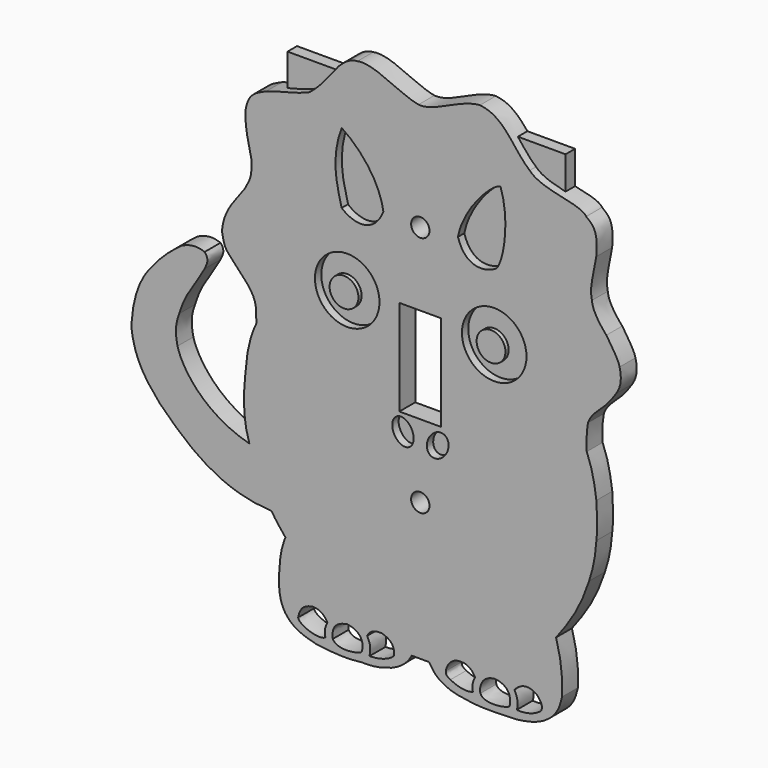
from build123d import *

# Parameters (mm, degrees)
F0_R     = 8.1256279654
F1_DEPTH = 5
F2_W     = 10.541
F2_H     = 24.0792
F2_R     = 2.3114
F3_DEPTH = 25
F2_R_2   = 8.1256279654
F4_DEPTH = 3
F5_DEPTH = 3
F6_R     = 3.6295881973
F7_DEPTH = 1


with BuildPart() as f1:
    # F0 (on Front) → F1 (new body)
    with BuildSketch(Plane.XZ):
        with BuildLine():
            add(Edge.make_bspline(
                [(-7.4735344388, 49.4673959911), (-3.9859429623, 52.6099316776), (-1.3800812885, 58.6650632322), (2.9892399907, 58.8950030506)],
                knots=[0, 0, 0, 0, 14.0836580344, 14.0836580344, 14.0836580344, 14.0836580344], degree=3))
            add(Edge.make_bspline(
                [(-9.6692116931, 47.8537157178), (-8.7991049513, 48.0954125524), (-8.2054268569, 48.9295025667), (-7.4735344388, 49.4673959911)],
                knots=[0, 0, 0, 0, 2.7248784615, 2.7248784615, 2.7248784615, 2.7248784615], degree=3))
            add(Edge.make_bspline(
                [(-19.9654772878, 44.760003686), (-16.485048458, 46.0168235004), (-12.5695681199, 46.5968959033), (-9.6692116931, 47.8537157178)],
                knots=[0, 0, 0, 0, 10.7510064334, 10.7510064334, 10.7510064334, 10.7510064334], degree=3))
            add(Edge.make_bspline(
                [(-25.1377783716, 38.9592945576), (-24.5093684644, 43.2614870369), (-22.0924057066, 43.6965376139), (-19.9654772878, 44.760003686)],
                knots=[0, 0, 0, 0, 7.7718031945, 7.7718031945, 7.7718031945, 7.7718031945], degree=3))
            add(Edge.make_bspline(
                [(-23.6875992268, 28.5180080682), (-24.6060471982, 32.530169934), (-25.3794752061, 35.7205606997), (-25.1377783716, 38.9592945576)],
                knots=[0, 0, 0, 0, 10.5415123728, 10.5415123728, 10.5415123728, 10.5415123728], degree=3))
            add(Edge.make_bspline(
                [(-25.3311358392, 21.4604754001), (-24.3643503636, 23.2973676175), (-23.397564888, 24.31249246), (-23.6875992268, 28.5180080682)],
                knots=[0, 0, 0, 0, 7.2463770229, 7.2463770229, 7.2463770229, 7.2463770229], degree=3))
            add(Edge.make_bspline(
                [(-31.083509326, 10.1490849629), (-30.7451337576, 15.321386978), (-27.4097230285, 18.3184221387), (-25.3311358392, 21.4604754001)],
                knots=[0, 0, 0, 0, 12.6900494228, 12.6900494228, 12.6900494228, 12.6900494228], degree=3))
            add(Edge.make_bspline(
                [(-25.0410996377, 0.9162835195), (-30.9384912252, 7.1520498022), (-30.310081318, 6.3302819617), (-31.083509326, 10.1490849629)],
                knots=[0, 0, 0, 0, 11.0342801004, 11.0342801004, 11.0342801004, 11.0342801004], degree=3))
            add(Edge.make_bspline(
                [(-22.4307794124, -7.494749967), (-22.4791187793, -4.4493759051), (-22.092403844, -2.3224479519), (-25.0410996377, 0.9162835195)],
                knots=[0, 0, 0, 0, 8.8067733018, 8.8067733018, 8.8067733018, 8.8067733018], degree=3))
            add(Edge.make_bspline(
                [(-24.6543865651, -14.6006224677), (-24.1709947586, -12.0869809762), (-23.4942436218, -9.5733385533), (-22.4307794124, -7.494749967)],
                knots=[0, 0, 0, 0, 7.4456599953, 7.4456599953, 7.4456599953, 7.4456599953], degree=3))
            add(Edge.make_bspline(
                [(-24.1888128221, -34.6901416779), (-26.3946000487, -28.0872806907), (-25.427814573, -21.4164610952), (-24.6543865651, -14.6006224677)],
                knots=[0, 0, 0, 0, 20.0949133117, 20.0949133117, 20.0949133117, 20.0949133117], degree=3))
            add(Edge.make_bspline(
                [(-42.2773174942, -18.9592409879), (-41.3830541074, -22.6988866925), (-36.2207144499, -31.3976258039), (-24.1888128221, -34.6901416779)],
                knots=[0, 0, 0, 0, 23.9719677496, 23.9719677496, 23.9719677496, 23.9719677496], degree=3))
            add(Edge.make_bspline(
                [(-41.8708324432, -11.6425445303), (-43.0902838707, -14.9757061154), (-42.7244491875, -16.7642310262), (-42.2773174942, -18.9592409879)],
                knots=[0, 0, 0, 0, 7.3279790631, 7.3279790631, 7.3279790631, 7.3279790631], degree=3))
            add(Edge.make_bspline(
                [(-35.4483984411, 0.3893578833), (-37.5892097751, -3.6212762546), (-40.3668470681, -6.439560093), (-41.8708324432, -11.6425445303)],
                knots=[0, 0, 0, 0, 13.6387072042, 13.6387072042, 13.6387072042, 13.6387072042], degree=3))
            add(Edge.make_bspline(
                [(-35.4483984411, 4.1290037334), (-34.2289470136, 2.7063123416), (-34.8386727273, 1.7714009155), (-35.4483984411, 0.3893578833)],
                knots=[0, 0, 0, 0, 3.7396458501, 3.7396458501, 3.7396458501, 3.7396458501], degree=3))
            add(Edge.make_bspline(
                [(-41.1798097193, 3.6818718072), (-38.4157262743, 4.9826181494), (-36.8304401636, 4.6167834662), (-35.4483984411, 4.1290037334)],
                knots=[0, 0, 0, 0, 5.7488261584, 5.7488261584, 5.7488261584, 5.7488261584], degree=3))
            add(Edge.make_bspline(
                [(-49.3359230459, -4.2219446041), (-46.992521733, -0.9926850908), (-44.5129722357, 1.2023242889), (-41.1798097193, 3.6818718072)],
                knots=[0, 0, 0, 0, 11.3574864499, 11.3574864499, 11.3574864499, 11.3574864499], degree=3))
            add(Edge.make_bspline(
                [(-53.9161786437, -18.1678049266), (-53.5743683577, -12.6304775476), (-52.275493741, -7.8451330774), (-49.3359230459, -4.2219446041)],
                knots=[0, 0, 0, 0, 14.6787520409, 14.6787520409, 14.6787520409, 14.6787520409], degree=3))
            add(Edge.make_bspline(
                [(-46.7602610588, -33.0900996923), (-50.1562654972, -29.1740968823), (-53.2325580716, -25.3458209336), (-53.9161786437, -18.1678049266)],
                knots=[0, 0, 0, 0, 16.5493817877, 16.5493817877, 16.5493817877, 16.5493817877], degree=3))
            add(Edge.make_bspline(
                [(-31.2933437526, -44.8141880333), (-37.0931662619, -42.1503633261), (-41.6853949428, -38.1865426898), (-46.7602610588, -33.0900996923)],
                knots=[0, 0, 0, 0, 19.408239961, 19.408239961, 19.408239961, 19.408239961], degree=3))
            add(Edge.make_bspline(
                [(-18.5950901359, -47.787938267), (-22.9360815138, -47.5999414921), (-26.9352607429, -46.745415777), (-31.2933437526, -44.8141880333)],
                knots=[0, 0, 0, 0, 13.0418110462, 13.0418110462, 13.0418110462, 13.0418110462], degree=3))
            add(Edge.make_bspline(
                [(-15.1086263359, -52.5390990078), (-16.2365995348, -51.0864071548), (-17.5696592778, -49.599532038), (-18.5950901359, -47.787938267)],
                knots=[0, 0, 0, 0, 5.8931280501, 5.8931280501, 5.8931280501, 5.8931280501], degree=3))
            add(Edge.make_bspline(
                [(-15.4485208914, -53.361248225), (-15.3352227062, -53.0871984859), (-15.221924521, -52.8131487469), (-15.1086263359, -52.5390990078)],
                knots=[0, 0, 0, 0, 0.8896390527, 0.8896390527, 0.8896390527, 0.8896390527], degree=3))
            add(Edge.make_bspline(
                [(-16.7295113206, -61.4822506905), (-16.5603235364, -58.7994158268), (-16.487814486, -56.3824549317), (-15.4485208914, -53.361248225)],
                knots=[0, 0, 0, 0, 8.2214121369, 8.2214121369, 8.2214121369, 8.2214121369], degree=3))
            add(Edge.make_bspline(
                [(-15.7143864781, -68.2739168406), (-16.6328325868, -66.3403496146), (-16.802020371, -63.8267025352), (-16.7295113206, -61.4822506905)],
                knots=[0, 0, 0, 0, 6.8671105671, 6.8671105671, 6.8671105671, 6.8671105671], degree=3))
            add(Edge.make_bspline(
                [(-7.2066746652, -73.6879184842), (-10.4454057291, -72.9386582971), (-13.950003311, -71.875192225), (-15.7143864781, -68.2739168406)],
                knots=[0, 0, 0, 0, 10.0842736024, 10.0842736024, 10.0842736024, 10.0842736024], degree=3))
            add(Edge.make_bspline(
                [(3.9551979862, -73.9692598581), (0, -74.5821967721), (-4.2821485549, -74.0021243691), (-7.2066746652, -73.6879184842)],
                knots=[0, 0, 0, 0, 11.1654177734, 11.1654177734, 11.1654177734, 11.1654177734], degree=3))
            add(Edge.make_bspline(
                [(11.6653125733, -72.7124512196), (9.2966873199, -73.5100358725), (7.6773217879, -74.0417689085), (3.9551979862, -73.9692598581)],
                knots=[0, 0, 0, 0, 7.8118778088, 7.8118778088, 7.8118778088, 7.8118778088], degree=3))
            add(Edge.make_bspline(
                [(16.6811458766, -68.3808848262), (15.4116060585, -70.7305371761), (13.743900694, -71.7940032482), (11.6653125733, -72.7124512196)],
                knots=[0, 0, 0, 0, 6.6272959152, 6.6272959152, 6.6272959152, 6.6272959152], degree=3))
            Line((16.6811458766, -68.3808848262), (21.055849269, -68.3808848262))
            add(Edge.make_bspline(
                [(24.2220722139, -71.740463376), (22.6027071476, -70.8945319057), (22.0468044281, -69.9035748839), (21.055849269, -68.3808848262)],
                knots=[0, 0, 0, 0, 4.6164635566, 4.6164635566, 4.6164635566, 4.6164635566], degree=3))
            add(Edge.make_bspline(
                [(32.125543803, -73.9399045706), (28.9593208581, -73.4565109015), (26.6148652881, -73.3356624842), (24.2220722139, -71.740463376)],
                knots=[0, 0, 0, 0, 8.2038042839, 8.2038042839, 8.2038042839, 8.2038042839], degree=3))
            add(Edge.make_bspline(
                [(43.1710705161, -73.9399045706), (39.6181307733, -74.0124136209), (35.6784798205, -74.3096638265), (32.125543803, -73.9399045706)],
                knots=[0, 0, 0, 0, 11.0455267131, 11.0455267131, 11.0455267131, 11.0455267131], degree=3))
            add(Edge.make_bspline(
                [(50.8612804115, -71.3768675923), (48.7300865352, -72.8764384985), (46.6031581163, -73.4806805849), (43.1710705161, -73.9399045706)],
                knots=[0, 0, 0, 0, 8.1060771515, 8.1060771515, 8.1060771515, 8.1060771515], degree=3))
            add(Edge.make_bspline(
                [(54.5201562345, -65.2140080929), (53.9505556226, -67.7998140454), (53.2188825309, -69.6289911866), (50.8612804115, -71.3768675923)],
                knots=[0, 0, 0, 0, 7.1671618859, 7.1671618859, 7.1671618859, 7.1671618859], degree=3))
            add(Edge.make_bspline(
                [(53.0161894858, -52.5328442454), (54.3150678277, -56.9763816893), (54.725240916, -60.9413795173), (54.5201562345, -65.2140080929)],
                knots=[0, 0, 0, 0, 12.7700365116, 12.7700365116, 12.7700365116, 12.7700365116], degree=3))
            add(Edge.make_bspline(
                [(61.3221749663, -37.3564660549), (59.1345913708, -44.1584922373), (56.2633872032, -48.2602156699), (53.0161894858, -52.5328442454)],
                knots=[0, 0, 0, 0, 17.3006314851, 17.3006314851, 17.3006314851, 17.3006314851], degree=3))
            add(Edge.make_bspline(
                [(63.1679520011, -27.7857780457), (62.8603249788, -31.9900475442), (62.313426286, -34.3143567443), (61.3221749663, -37.3564660549)],
                knots=[0, 0, 0, 0, 9.7470488781, 9.7470488781, 9.7470488781, 9.7470488781], degree=3))
            add(Edge.make_bspline(
                [(63.1679520011, -18.8645292073), (63.3046776056, -22.2484506667), (63.5439455509, -24.9145701528), (63.1679520011, -27.7857780457)],
                knots=[0, 0, 0, 0, 8.9212488383, 8.9212488383, 8.9212488383, 8.9212488383], degree=3))
            add(Edge.make_bspline(
                [(60.7411041856, -8.84948764), (62.142521143, -12.1650481597), (62.6894161105, -15.2413407341), (63.1679520011, -18.8645292073)],
                knots=[0, 0, 0, 0, 10.3048846629, 10.3048846629, 10.3048846629, 10.3048846629], degree=3))
            add(Edge.make_bspline(
                [(61.0487349331, -2.3550926708), (60.5701990426, -4.7819456086), (60.7069246471, -6.7986263894), (60.7411041856, -8.84948764)],
                knots=[0, 0, 0, 0, 6.5016769139, 6.5016769139, 6.5016769139, 6.5016769139], degree=3))
            add(Edge.make_bspline(
                [(64.0224814415, 1.5757256187), (62.9628747702, 0.5502947606), (61.7323555052, -0.4409550456), (61.0487349331, -2.3550926708)],
                knots=[0, 0, 0, 0, 4.9289451936, 4.9289451936, 4.9289451936, 4.9289451936], degree=3))
            add(Edge.make_bspline(
                [(68.1925714016, 6.4977942966), (66.9278725982, 4.5152939856), (65.628990531, 3.0113288667), (64.0224814415, 1.5757256187)],
                knots=[0, 0, 0, 0, 6.4510782312, 6.4510782312, 6.4510782312, 6.4510782312], degree=3))
            add(Edge.make_bspline(
                [(69.0129101276, 12.6161985099), (69.593988359, 10.0868018344), (69.3547204137, 8.3093885332), (68.1925714016, 6.4977942966)],
                knots=[0, 0, 0, 0, 6.1731536303, 6.1731536303, 6.1731536303, 6.1731536303], degree=3))
            add(Edge.make_bspline(
                [(65.6831264496, 18.5696575791), (66.8332402905, 16.5977720171), (68.4318318963, 14.7354220971), (69.0129101276, 12.6161985099)],
                knots=[0, 0, 0, 0, 6.821373339, 6.821373339, 6.821373339, 6.821373339], degree=3))
            add(Edge.make_bspline(
                [(62.0391406119, 25.0980686396), (62.1873699129, 22.8377301246), (64.2604380846, 20.114293322), (65.6831264496, 18.5696575791)],
                knots=[0, 0, 0, 0, 7.4765489205, 7.4765489205, 7.4765489205, 7.4765489205], degree=3))
            add(Edge.make_bspline(
                [(63.1329342723, 35.1472906768), (62.2442252934, 29.815049842), (61.4238828421, 28.1060002744), (62.0391406119, 25.0980686396)],
                knots=[0, 0, 0, 0, 10.1085730014, 10.1085730014, 10.1085730014, 10.1085730014], degree=3))
            add(Edge.make_bspline(
                [(60.6035366654, 43.2140156627), (61.9707778096, 41.9834963977), (63.7481957674, 41.3682386279), (63.1329342723, 35.1472906768)],
                knots=[0, 0, 0, 0, 8.4539874764, 8.4539874764, 8.4539874764, 8.4539874764], degree=3))
            add(Edge.make_bspline(
                [(46.3709793985, 48.8015934825), (49.7339703143, 45.3332364559), (58.9628480375, 45.6750504673), (60.6035366654, 43.2140156627)],
                knots=[0, 0, 0, 0, 15.2900854232, 15.2900854232, 15.2900854232, 15.2900854232], degree=3))
            add(Edge.make_bspline(
                [(33.8607244194, 59.1926276684), (40.0816723704, 58.5773661733), (42.2008944054, 52.2652715445), (46.3709793985, 48.8015934825)],
                knots=[0, 0, 0, 0, 16.262843266, 16.262843266, 16.262843266, 16.262843266], degree=3))
            add(Edge.make_bspline(
                [(18.3949004859, 54.29616943), (22.5126221776, 53.8603849709), (28.8019310683, 58.9191801846), (33.8607244194, 59.1926276684)],
                knots=[0, 0, 0, 0, 16.2224231612, 16.2224231612, 16.2224231612, 16.2224231612], degree=3))
            add(Edge.make_bspline(
                [(2.9892399907, 58.8950030506), (7.3577007279, 59.7848258913), (13.6810950935, 55.1009662449), (18.3949004859, 54.29616943)],
                knots=[0, 0, 0, 0, 16.0774265964, 16.0774265964, 16.0774265964, 16.0774265964], degree=3))
        make_face()
        with BuildLine():
            add(Edge.make_bspline(
                [(-5.0339726731, -71.4123174548), (-6.8113859743, -72.6428329945), (-11.870178394, -70.5919712782), (-11.9043597952, -69.224730134)],
                knots=[0, 0, 0, 0, 7.2102536358, 7.2102536358, 7.2102536358, 7.2102536358], degree=3))
            add(Edge.make_bspline(
                [(-11.9043597952, -69.224730134), (-11.5967299789, -67.6524043083), (-11.04983408, -66.0117194057), (-8.1786271185, -65.6357258558)],
                knots=[0, 0, 0, 0, 5.1732036193, 5.1732036193, 5.1732036193, 5.1732036193], degree=3))
            add(Edge.make_bspline(
                [(-8.1786271185, -65.6357258558), (-8.0988714471, -65.6357258558), (-8.0191157758, -65.6357258558), (-7.9393601045, -65.6357258558)],
                knots=[0, 0, 0, 0, 0.239267014, 0.239267014, 0.239267014, 0.239267014], degree=3))
            add(Edge.make_bspline(
                [(-7.9393601045, -65.6357258558), (-6.8113859743, -65.7724514604), (-5.4783262312, -66.1142617464), (-4.5554381795, -67.9600313306)],
                knots=[0, 0, 0, 0, 4.1052799581, 4.1052799581, 4.1052799581, 4.1052799581], degree=3))
            add(Edge.make_bspline(
                [(-4.5554381795, -67.9600313306), (-5.3757829592, -69.6007236838), (-5.2732401527, -70.4894289374), (-5.0339726731, -71.4123174548)],
                knots=[0, 0, 0, 0, 3.4852940687, 3.4852940687, 3.4852940687, 3.4852940687], degree=3))
        make_face(mode=Mode.SUBTRACT)
        with BuildLine():
            add(Edge.make_bspline(
                [(-3.1881972682, -71.1388736963), (-2.060223138, -73.5657215118), (4.3999911286, -72.1984803677), (4.092361778, -71.5148597956)],
                knots=[0, 0, 0, 0, 7.2902610085, 7.2902610085, 7.2902610085, 7.2902610085], degree=3))
            add(Edge.make_bspline(
                [(-3.1881972682, -71.1388736963), (-3.8034557365, -67.1396926045), (-0.2828098659, -66.9004246593), (0.434991729, -66.6953399777)],
                knots=[0, 0, 0, 0, 5.7334536204, 5.7334536204, 5.7334536204, 5.7334536204], degree=3))
            add(Edge.make_bspline(
                [(0.434991729, -66.6953399777), (5.1861549728, -67.3105940223), (4.3316292576, -71.1730495095), (4.092361778, -71.5148597956)],
                knots=[0, 0, 0, 0, 6.0501344572, 6.0501344572, 6.0501344572, 6.0501344572], degree=3))
        make_face(mode=Mode.SUBTRACT)
        with BuildLine():
            add(Edge.make_bspline(
                [(6.0748616233, -71.9250366092), (8.6384387687, -71.9592124224), (11.270377785, -71.036323905), (12.1932663023, -69.8741748929)],
                knots=[0, 0, 0, 0, 6.4529768011, 6.4529768011, 6.4529768011, 6.4529768011], degree=3))
            add(Edge.make_bspline(
                [(5.4596033879, -67.6524043083), (6.0406806879, -68.8487440348), (6.4508528449, -69.3272724748), (6.0748616233, -71.9250366092)],
                knots=[0, 0, 0, 0, 4.3167035426, 4.3167035426, 4.3167035426, 4.3167035426], degree=3))
            add(Edge.make_bspline(
                [(9.0486109257, -65.8408105373), (7.6130079105, -65.8749938011), (6.314129103, -65.9775361419), (5.4596033879, -67.6524043083)],
                knots=[0, 0, 0, 0, 4.0203043538, 4.0203043538, 4.0203043538, 4.0203043538], degree=3))
            add(Edge.make_bspline(
                [(12.1932663023, -69.8741748929), (12.1590849012, -69.224730134), (12.7743436024, -66.8320581317), (9.0486109257, -65.8408105373)],
                knots=[0, 0, 0, 0, 5.1143802618, 5.1143802618, 5.1143802618, 5.1143802618], degree=3))
        make_face(mode=Mode.SUBTRACT)
        with BuildLine():
            add(Edge.make_bspline(
                [(25.2845995128, -68.9854621887), (25.1274835318, -69.9679404497), (25.9820092469, -70.2926591039), (26.4263637364, -70.549018681)],
                knots=[0, 0, 0, 0, 1.9360615814, 1.9360615814, 1.9360615814, 1.9360615814], degree=3))
            add(Edge.make_bspline(
                [(25.2845995128, -68.9854621887), (25.2504181117, -68.4385672212), (26.2074880302, -65.2939155698), (29.6255908906, -65.7382681966)],
                knots=[0, 0, 0, 0, 5.4211138122, 5.4211138122, 5.4211138122, 5.4211138122], degree=3))
            add(Edge.make_bspline(
                [(29.6255908906, -65.7382681966), (30.2066672593, -65.7040849328), (31.8473577499, -66.3193464279), (32.6335206628, -68.0283978581)],
                knots=[0, 0, 0, 0, 3.7805205172, 3.7805205172, 3.7805205172, 3.7805205172], degree=3))
            add(Edge.make_bspline(
                [(32.6335206628, -68.0283978581), (32.2233475745, -68.6436519027), (31.6764526069, -70.1818019152), (32.1208052337, -71.4465007186)],
                knots=[0, 0, 0, 0, 3.4563426155, 3.4563426155, 3.4563426155, 3.4563426155], degree=3))
            add(Edge.make_bspline(
                [(26.4263637364, -70.549018681), (28.6139491946, -71.6940835118), (30.510995537, -71.8991681933), (32.1208052337, -71.4465007186)],
                knots=[0, 0, 0, 0, 5.7647322552, 5.7647322552, 5.7647322552, 5.7647322552], degree=3))
        make_face(mode=Mode.SUBTRACT)
        with BuildLine():
            add(Edge.make_bspline(
                [(33.9803695679, -71.1300969124), (34.9203497171, -73.5056772828), (41.9103689492, -72.1384361386), (41.3463823497, -71.3522732258)],
                knots=[0, 0, 0, 0, 7.3693627009, 7.3693627009, 7.3693627009, 7.3693627009], degree=3))
            add(Edge.make_bspline(
                [(33.9803695679, -71.1300969124), (33.6898304522, -70.1046660542), (33.9290983975, -66.9770985842), (37.7061031759, -66.7207464576)],
                knots=[0, 0, 0, 0, 5.7726477765, 5.7726477765, 5.7726477765, 5.7726477765], degree=3))
            add(Edge.make_bspline(
                [(37.7061031759, -66.7207464576), (41.9958233833, -67.2334581614), (41.5001958609, -70.617377758), (41.3463823497, -71.3522732258)],
                knots=[0, 0, 0, 0, 5.8908974417, 5.8908974417, 5.8908974417, 5.8908974417], degree=3))
        make_face(mode=Mode.SUBTRACT)
        with BuildLine():
            add(Edge.make_bspline(
                [(42.5085350871, -67.5239935517), (43.0212505162, -68.3785229921), (43.7390506268, -70.2243000269), (43.106701225, -71.8137174845)],
                knots=[0, 0, 0, 0, 4.3312277876, 4.3312277876, 4.3312277876, 4.3312277876], degree=3))
            add(Edge.make_bspline(
                [(42.5085350871, -67.5239935517), (42.9187044501, -67.1309158206), (45.2942885458, -64.3280670047), (48.4902150929, -67.0796409249)],
                knots=[0, 0, 0, 0, 5.9981617975, 5.9981617975, 5.9981617975, 5.9981617975], degree=3))
            add(Edge.make_bspline(
                [(48.4902150929, -67.0796409249), (49.1225644946, -67.9341703653), (49.9599985778, -69.0792351961), (49.0883812308, -70.207208395)],
                knots=[0, 0, 0, 0, 3.1842551733, 3.1842551733, 3.1842551733, 3.1842551733], degree=3))
            add(Edge.make_bspline(
                [(49.0883812308, -70.207208395), (47.4135130644, -71.3693648577), (45.6873700023, -71.9675272703), (43.106701225, -71.8137174845)],
                knots=[0, 0, 0, 0, 6.1936553945, 6.1936553945, 6.1936553945, 6.1936553945], degree=3))
        make_face(mode=Mode.SUBTRACT)
        with BuildLine():
            add(Edge.make_bspline(
                [(13.104589656, -16.4676252753), (9.1005951627, -18.287623223), (13.1534541256, -21.8895189073), (17.2063130885, -25.4914145917), (17.1574486189, -20.0695209596), (17.1085841493, -14.6476273275), (13.104589656, -16.4676252753)],
                knots=[0, 0, 0, 2.0943951024, 2.0943951024, 4.1887902048, 4.1887902048, 6.2831853072, 6.2831853072, 6.2831853072], degree=2, weights=[1, 0.5, 1, 0.5, 1, 0.5, 1]))
        make_face(mode=Mode.SUBTRACT)
        with BuildLine():
            add(Edge.make_bspline(
                [(25.0679496676, -16.8777965009), (21.5726752041, -14.5760314673), (20.5516496777, -19.93118162), (19.5306241512, -25.2863317728), (24.0469241411, -22.2329466537), (28.563224131, -19.1795615346), (25.0679496676, -16.8777965009)],
                knots=[0, 0, 0, 2.0943951024, 2.0943951024, 4.1887902048, 4.1887902048, 6.2831853072, 6.2831853072, 6.2831853072], degree=2, weights=[1, 0.5, 1, 0.5, 1, 0.5, 1]))
        make_face(mode=Mode.SUBTRACT)
        with BuildLine():
            add(Edge.make_bspline(
                [(18.8032221049, -2.7508533094), (16.9334001839, -6.0027190484), (15.3074664995, -9.010694921), (15.957839787, -12.7909891307)],
                knots=[0, 0, 0, 0, 10.4355415694, 10.4355415694, 10.4355415694, 10.4355415694], degree=3))
            add(Edge.make_bspline(
                [(18.8032221049, -2.7508533094), (20.6730458885, -5.5962358601), (22.2176816314, -8.4416186437), (21.8518469483, -12.6690436155)],
                knots=[0, 0, 0, 0, 10.376155954, 10.376155954, 10.376155954, 10.376155954], degree=3))
            add(Edge.make_bspline(
                [(15.957839787, -12.7909891307), (19.1690567881, -16.083503142), (21.0795290768, -13.5633070022), (21.8518469483, -12.6690436155)],
                knots=[0, 0, 0, 0, 5.8952685372, 5.8952685372, 5.8952685372, 5.8952685372], degree=3))
        make_face(mode=Mode.SUBTRACT)
        with Locations((0.434991729, 7.2993612848)):
            Circle(F0_R, mode=Mode.SUBTRACT)
        with BuildLine():
            add(Edge.make_bspline(
                [(-0.953837065, 42.8298301995), (-3.9618131705, 35.0253507495), (-1.8481005682, 28.6842118949), (-0.953837065, 25.1071602106)],
                knots=[0, 0, 0, 0, 17.7226699889, 17.7226699889, 17.7226699889, 17.7226699889], degree=3))
            add(Edge.make_bspline(
                [(-0.953837065, 42.8298301995), (2.867105417, 40.3909273446), (8.3952769637, 34.8627567291), (9.5334304497, 27.7086533606)],
                knots=[0, 0, 0, 0, 18.40197731, 18.40197731, 18.40197731, 18.40197731], degree=3))
            add(Edge.make_bspline(
                [(-0.953837065, 25.1071602106), (1.8915452529, 22.5869640708), (7.1758273989, 21.6114036739), (9.5334304497, 27.7086533606)],
                knots=[0, 0, 0, 0, 10.805116683, 10.805116683, 10.805116683, 10.805116683], degree=3))
        make_face(mode=Mode.SUBTRACT)
        with Locations((37.4433604186, 7.2993614193)):
            Circle(F0_R, mode=Mode.SUBTRACT)
        with BuildLine():
            add(Edge.make_bspline(
                [(39.0441119671, 42.8298301995), (37.1742881835, 42.9111234844), (29.6949986368, 35.5131290853), (28.3129550517, 28.1964316964)],
                knots=[0, 0, 0, 0, 18.1464619277, 18.1464619277, 18.1464619277, 18.1464619277], degree=3))
            add(Edge.make_bspline(
                [(39.0441119671, 42.8298301995), (41.5643081069, 35.3505387902), (39.6131873131, 25.9201265872), (37.9872582853, 24.3754889816)],
                knots=[0, 0, 0, 0, 18.4845786939, 18.4845786939, 18.4845786939, 18.4845786939], degree=3))
            add(Edge.make_bspline(
                [(28.3129550517, 28.1964316964), (30.5079650134, 21.1236253381), (36.3613218069, 23.1560412794), (37.9872582853, 24.3754889816)],
                knots=[0, 0, 0, 0, 10.4015261518, 10.4015261518, 10.4015261518, 10.4015261518], degree=3))
        make_face(mode=Mode.SUBTRACT)
    extrude(amount=F1_DEPTH)

    # F2 (on face) → F3 (cut)
    with BuildSketch(Plane(origin=(0, 0, 0), x_dir=(-1, 0, 0), z_dir=(0, 1, 0))):
        with Locations((-18.8377820528, -3.2537430525)):
            Rectangle(F2_W, F2_H)
        with BuildLine():
            add(Edge.make_bspline(
                [(-18.8032221049, -2.7508533094), (-20.6730458885, -5.5962358601), (-22.2176816314, -8.4416186437), (-21.8518469483, -12.6690436155)],
                knots=[0, 0, 0, 0, 10.376155954, 10.376155954, 10.376155954, 10.376155954], degree=3))
            add(Edge.make_bspline(
                [(-18.8032221049, -2.7508533094), (-16.9334001839, -6.0027190484), (-15.3074664995, -9.010694921), (-15.957839787, -12.7909891307)],
                knots=[0, 0, 0, 0, 10.4355415694, 10.4355415694, 10.4355415694, 10.4355415694], degree=3))
            add(Edge.make_bspline(
                [(-15.957839787, -12.7909891307), (-19.1690567881, -16.083503142), (-21.0795290768, -13.5633070022), (-21.8518469483, -12.6690436155)],
                knots=[0, 0, 0, 0, 5.8952685372, 5.8952685372, 5.8952685372, 5.8952685372], degree=3))
        make_face(mode=Mode.SUBTRACT)
        with Locations((-18.8377820528, 27.2262569475)):
            Circle(F2_R)
        with Locations((-18.8377820528, -33.7337430525)):
            Circle(F2_R)
    extrude(amount=-F3_DEPTH, mode=Mode.SUBTRACT)

    # F2 (on face) → F4 (join)
    with BuildSketch(Plane(origin=(0, 0, 0), x_dir=(-1, 0, 0), z_dir=(0, 1, 0))):
        with BuildLine():
            Line((-53.7984021581, 45.705300692), (-53.7984021581, -3.2537430525))
            Line((-53.7984021581, -3.2537430525), (-53.7984021581, -51.4954857945))
            add(Edge.make_bspline(
                [(-53.7984021581, -51.4954857945), (-53.5402452993, -51.8411686296), (-53.279453097, -52.186444757), (-53.0161894858, -52.5328442454)],
                knots=[15.8979984715, 15.8979984715, 15.8979984715, 15.8979984715, 17.3006314851, 17.3006314851, 17.3006314851, 17.3006314851], degree=3))
            add(Edge.make_bspline(
                [(-53.0161894858, -52.5328442454), (-53.3263659796, -53.5939758543), (-53.5858622452, -54.6278177662), (-53.7984021581, -55.6450762439)],
                knots=[0, 0, 0, 0, 3.0495274451, 3.0495274451, 3.0495274451, 3.0495274451], degree=3))
            Line((-53.7984021581, -55.6450762439), (-53.7984021581, -60.4894645512))
            Line((-53.7984021581, -60.4894645512), (16.1898299479, -60.4894645512))
            Line((16.1898299479, -60.4894645512), (16.1898299479, -56.1341148175))
            add(Edge.make_bspline(
                [(16.1898299479, -56.1341148175), (16.0199518066, -55.2534494979), (15.784864082, -54.3389914811), (15.4485208914, -53.361248225)],
                knots=[5.5607433866, 5.5607433866, 5.5607433866, 5.5607433866, 8.2214121369, 8.2214121369, 8.2214121369, 8.2214121369], degree=3))
            add(Edge.make_bspline(
                [(15.4485208914, -53.361248225), (15.3352227062, -53.0871984859), (15.221924521, -52.8131487469), (15.1086263359, -52.5390990078)],
                knots=[0, 0, 0, 0, 0.8896390527, 0.8896390527, 0.8896390527, 0.8896390527], degree=3))
            add(Edge.make_bspline(
                [(15.1086263359, -52.5390990078), (15.454660807, -52.0934488296), (15.8199962125, -51.6445816245), (16.1898299479, -51.1841093467)],
                knots=[0, 0, 0, 0, 1.8078669335, 1.8078669335, 1.8078669335, 1.8078669335], degree=3))
            Line((16.1898299479, -51.1841093467), (16.1898299479, -3.2537430525))
            Line((16.1898299479, -3.2537430525), (16.1898299479, 45.8951678371))
            add(Edge.make_bspline(
                [(16.1898299479, 45.8951678371), (13.8531123489, 46.5093258284), (11.5481471026, 47.0395112184), (9.6692116931, 47.8537157178)],
                knots=[3.7861911823, 3.7861911823, 3.7861911823, 3.7861911823, 10.7510064334, 10.7510064334, 10.7510064334, 10.7510064334], degree=3))
            add(Edge.make_bspline(
                [(9.6692116931, 47.8537157178), (8.7991049513, 48.0954125524), (8.2054268569, 48.9295025667), (7.4735344388, 49.4673959911)],
                knots=[0, 0, 0, 0, 2.7248784615, 2.7248784615, 2.7248784615, 2.7248784615], degree=3))
            add(Edge.make_bspline(
                [(7.4735344388, 49.4673959911), (6.1056557778, 50.6999392909), (4.8734145161, 52.3805301988), (3.6172144063, 53.9819784462)],
                knots=[0, 0, 0, 0, 5.5237935475, 5.5237935475, 5.5237935475, 5.5237935475], degree=3))
            Line((3.6172144063, 53.9819784462), (-41.793309606, 53.9819784462))
            add(Edge.make_bspline(
                [(-41.793309606, 53.9819784462), (-43.2593832227, 52.172105367), (-44.6381098487, 50.2409172022), (-46.3709793985, 48.8015934825)],
                knots=[9.5048548953, 9.5048548953, 9.5048548953, 9.5048548953, 16.262843266, 16.262843266, 16.262843266, 16.262843266], degree=3))
            add(Edge.make_bspline(
                [(-46.3709793985, 48.8015934825), (-47.9886629733, 47.133226147), (-50.9636265231, 46.3464763778), (-53.7984021581, 45.705300692)],
                knots=[0, 0, 0, 0, 7.3549172941, 7.3549172941, 7.3549172941, 7.3549172941], degree=3))
        make_face()
        with Locations((-18.8377820528, -33.7337430525)):
            Circle(F2_R, mode=Mode.SUBTRACT)
        with BuildLine():
            add(Edge.make_bspline(
                [(-25.0679496676, -16.8777965009), (-21.5726752041, -14.5760314673), (-20.5516496777, -19.93118162), (-19.5306241512, -25.2863317728), (-24.0469241411, -22.2329466537), (-28.563224131, -19.1795615346), (-25.0679496676, -16.8777965009)],
                knots=[0, 0, 0, 2.0943951024, 2.0943951024, 4.1887902048, 4.1887902048, 6.2831853072, 6.2831853072, 6.2831853072], degree=2, weights=[1, 0.5, 1, 0.5, 1, 0.5, 1]))
        make_face(mode=Mode.SUBTRACT)
        with BuildLine():
            add(Edge.make_bspline(
                [(-13.104589656, -16.4676252753), (-9.1005951627, -18.287623223), (-13.1534541256, -21.8895189073), (-17.2063130885, -25.4914145917), (-17.1574486189, -20.0695209596), (-17.1085841493, -14.6476273275), (-13.104589656, -16.4676252753)],
                knots=[0, 0, 0, 2.0943951024, 2.0943951024, 4.1887902048, 4.1887902048, 6.2831853072, 6.2831853072, 6.2831853072], degree=2, weights=[1, 0.5, 1, 0.5, 1, 0.5, 1]))
        make_face(mode=Mode.SUBTRACT)
        with Locations((-37.4433604186, 7.2993614193)):
            Circle(F2_R_2, mode=Mode.SUBTRACT)
        with Locations((-18.8377820528, -3.2537430525)):
            Rectangle(F2_W, F2_H, mode=Mode.SUBTRACT)
        with BuildLine():
            add(Edge.make_bspline(
                [(-39.0441119671, 42.8298301995), (-41.5643081069, 35.3505387902), (-39.6131873131, 25.9201265872), (-37.9872582853, 24.3754889816)],
                knots=[0, 0, 0, 0, 18.4845786939, 18.4845786939, 18.4845786939, 18.4845786939], degree=3))
            add(Edge.make_bspline(
                [(-39.0441119671, 42.8298301995), (-37.1742881835, 42.9111234844), (-29.6949986368, 35.5131290853), (-28.3129550517, 28.1964316964)],
                knots=[0, 0, 0, 0, 18.1464619277, 18.1464619277, 18.1464619277, 18.1464619277], degree=3))
            add(Edge.make_bspline(
                [(-28.3129550517, 28.1964316964), (-30.5079650134, 21.1236253381), (-36.3613218069, 23.1560412794), (-37.9872582853, 24.3754889816)],
                knots=[0, 0, 0, 0, 10.4015261518, 10.4015261518, 10.4015261518, 10.4015261518], degree=3))
        make_face(mode=Mode.SUBTRACT)
        with Locations((-18.8377820528, 27.2262569475)):
            Circle(F2_R, mode=Mode.SUBTRACT)
        with Locations((-0.434991729, 7.2993612848)):
            Circle(F2_R_2, mode=Mode.SUBTRACT)
        with BuildLine():
            add(Edge.make_bspline(
                [(0.953837065, 42.8298301995), (-2.867105417, 40.3909273446), (-8.3952769637, 34.8627567291), (-9.5334304497, 27.7086533606)],
                knots=[0, 0, 0, 0, 18.40197731, 18.40197731, 18.40197731, 18.40197731], degree=3))
            add(Edge.make_bspline(
                [(0.953837065, 42.8298301995), (3.9618131705, 35.0253507495), (1.8481005682, 28.6842118949), (0.953837065, 25.1071602106)],
                knots=[0, 0, 0, 0, 17.7226699889, 17.7226699889, 17.7226699889, 17.7226699889], degree=3))
            add(Edge.make_bspline(
                [(0.953837065, 25.1071602106), (-1.8915452529, 22.5869640708), (-7.1758273989, 21.6114036739), (-9.5334304497, 27.7086533606)],
                knots=[0, 0, 0, 0, 10.805116683, 10.805116683, 10.805116683, 10.805116683], degree=3))
        make_face(mode=Mode.SUBTRACT)
        with BuildLine():
            Line((-53.7984021581, 53.9819784462), (-53.7984021581, 45.705300692))
            add(Edge.make_bspline(
                [(-46.3709793985, 48.8015934825), (-47.9886629733, 47.133226147), (-50.9636265231, 46.3464763778), (-53.7984021581, 45.705300692)],
                knots=[0, 0, 0, 0, 7.3549172941, 7.3549172941, 7.3549172941, 7.3549172941], degree=3))
            add(Edge.make_bspline(
                [(-41.793309606, 53.9819784462), (-43.2593832227, 52.172105367), (-44.6381098487, 50.2409172022), (-46.3709793985, 48.8015934825)],
                knots=[9.5048548953, 9.5048548953, 9.5048548953, 9.5048548953, 16.262843266, 16.262843266, 16.262843266, 16.262843266], degree=3))
            Line((-41.793309606, 53.9819784462), (-53.7984021581, 53.9819784462))
        make_face()
        with BuildLine():
            Line((16.1898299479, 53.9819784462), (3.6172144063, 53.9819784462))
            add(Edge.make_bspline(
                [(7.4735344388, 49.4673959911), (6.1056557778, 50.6999392909), (4.8734145161, 52.3805301988), (3.6172144063, 53.9819784462)],
                knots=[0, 0, 0, 0, 5.5237935475, 5.5237935475, 5.5237935475, 5.5237935475], degree=3))
            add(Edge.make_bspline(
                [(9.6692116931, 47.8537157178), (8.7991049513, 48.0954125524), (8.2054268569, 48.9295025667), (7.4735344388, 49.4673959911)],
                knots=[0, 0, 0, 0, 2.7248784615, 2.7248784615, 2.7248784615, 2.7248784615], degree=3))
            add(Edge.make_bspline(
                [(16.1898299479, 45.8951678371), (13.8531123489, 46.5093258284), (11.5481471026, 47.0395112184), (9.6692116931, 47.8537157178)],
                knots=[3.7861911823, 3.7861911823, 3.7861911823, 3.7861911823, 10.7510064334, 10.7510064334, 10.7510064334, 10.7510064334], degree=3))
            Line((16.1898299479, 45.8951678371), (16.1898299479, 53.9819784462))
        make_face()
        with Locations((-0.434991729, 7.2993612848)):
            Circle(F2_R_2)
        with Locations((-37.4433604186, 7.2993614193)):
            Circle(F2_R_2)
    extrude(amount=-F4_DEPTH)

    # F2 (on face) → F5 (join)
    with BuildSketch(Plane(origin=(0, 0, 0), x_dir=(-1, 0, 0), z_dir=(0, 1, 0))):
        with BuildLine():
            Line((-53.7984021581, 45.705300692), (-53.7984021581, -3.2537430525))
            Line((-53.7984021581, -3.2537430525), (-53.7984021581, -51.4954857945))
            add(Edge.make_bspline(
                [(-53.7984021581, -51.4954857945), (-53.5402452993, -51.8411686296), (-53.279453097, -52.186444757), (-53.0161894858, -52.5328442454)],
                knots=[15.8979984715, 15.8979984715, 15.8979984715, 15.8979984715, 17.3006314851, 17.3006314851, 17.3006314851, 17.3006314851], degree=3))
            add(Edge.make_bspline(
                [(-53.0161894858, -52.5328442454), (-53.3263659796, -53.5939758543), (-53.5858622452, -54.6278177662), (-53.7984021581, -55.6450762439)],
                knots=[0, 0, 0, 0, 3.0495274451, 3.0495274451, 3.0495274451, 3.0495274451], degree=3))
            Line((-53.7984021581, -55.6450762439), (-53.7984021581, -60.4894645512))
            Line((-53.7984021581, -60.4894645512), (16.1898299479, -60.4894645512))
            Line((16.1898299479, -60.4894645512), (16.1898299479, -56.1341148175))
            add(Edge.make_bspline(
                [(16.1898299479, -56.1341148175), (16.0199518066, -55.2534494979), (15.784864082, -54.3389914811), (15.4485208914, -53.361248225)],
                knots=[5.5607433866, 5.5607433866, 5.5607433866, 5.5607433866, 8.2214121369, 8.2214121369, 8.2214121369, 8.2214121369], degree=3))
            add(Edge.make_bspline(
                [(15.4485208914, -53.361248225), (15.3352227062, -53.0871984859), (15.221924521, -52.8131487469), (15.1086263359, -52.5390990078)],
                knots=[0, 0, 0, 0, 0.8896390527, 0.8896390527, 0.8896390527, 0.8896390527], degree=3))
            add(Edge.make_bspline(
                [(15.1086263359, -52.5390990078), (15.454660807, -52.0934488296), (15.8199962125, -51.6445816245), (16.1898299479, -51.1841093467)],
                knots=[0, 0, 0, 0, 1.8078669335, 1.8078669335, 1.8078669335, 1.8078669335], degree=3))
            Line((16.1898299479, -51.1841093467), (16.1898299479, -3.2537430525))
            Line((16.1898299479, -3.2537430525), (16.1898299479, 45.8951678371))
            add(Edge.make_bspline(
                [(16.1898299479, 45.8951678371), (13.8531123489, 46.5093258284), (11.5481471026, 47.0395112184), (9.6692116931, 47.8537157178)],
                knots=[3.7861911823, 3.7861911823, 3.7861911823, 3.7861911823, 10.7510064334, 10.7510064334, 10.7510064334, 10.7510064334], degree=3))
            add(Edge.make_bspline(
                [(9.6692116931, 47.8537157178), (8.7991049513, 48.0954125524), (8.2054268569, 48.9295025667), (7.4735344388, 49.4673959911)],
                knots=[0, 0, 0, 0, 2.7248784615, 2.7248784615, 2.7248784615, 2.7248784615], degree=3))
            add(Edge.make_bspline(
                [(7.4735344388, 49.4673959911), (6.1056557778, 50.6999392909), (4.8734145161, 52.3805301988), (3.6172144063, 53.9819784462)],
                knots=[0, 0, 0, 0, 5.5237935475, 5.5237935475, 5.5237935475, 5.5237935475], degree=3))
            Line((3.6172144063, 53.9819784462), (-41.793309606, 53.9819784462))
            add(Edge.make_bspline(
                [(-41.793309606, 53.9819784462), (-43.2593832227, 52.172105367), (-44.6381098487, 50.2409172022), (-46.3709793985, 48.8015934825)],
                knots=[9.5048548953, 9.5048548953, 9.5048548953, 9.5048548953, 16.262843266, 16.262843266, 16.262843266, 16.262843266], degree=3))
            add(Edge.make_bspline(
                [(-46.3709793985, 48.8015934825), (-47.9886629733, 47.133226147), (-50.9636265231, 46.3464763778), (-53.7984021581, 45.705300692)],
                knots=[0, 0, 0, 0, 7.3549172941, 7.3549172941, 7.3549172941, 7.3549172941], degree=3))
        make_face()
        with Locations((-18.8377820528, -33.7337430525)):
            Circle(F2_R, mode=Mode.SUBTRACT)
        with BuildLine():
            add(Edge.make_bspline(
                [(-25.0679496676, -16.8777965009), (-21.5726752041, -14.5760314673), (-20.5516496777, -19.93118162), (-19.5306241512, -25.2863317728), (-24.0469241411, -22.2329466537), (-28.563224131, -19.1795615346), (-25.0679496676, -16.8777965009)],
                knots=[0, 0, 0, 2.0943951024, 2.0943951024, 4.1887902048, 4.1887902048, 6.2831853072, 6.2831853072, 6.2831853072], degree=2, weights=[1, 0.5, 1, 0.5, 1, 0.5, 1]))
        make_face(mode=Mode.SUBTRACT)
        with BuildLine():
            add(Edge.make_bspline(
                [(-13.104589656, -16.4676252753), (-9.1005951627, -18.287623223), (-13.1534541256, -21.8895189073), (-17.2063130885, -25.4914145917), (-17.1574486189, -20.0695209596), (-17.1085841493, -14.6476273275), (-13.104589656, -16.4676252753)],
                knots=[0, 0, 0, 2.0943951024, 2.0943951024, 4.1887902048, 4.1887902048, 6.2831853072, 6.2831853072, 6.2831853072], degree=2, weights=[1, 0.5, 1, 0.5, 1, 0.5, 1]))
        make_face(mode=Mode.SUBTRACT)
        with Locations((-37.4433604186, 7.2993614193)):
            Circle(F2_R_2, mode=Mode.SUBTRACT)
        with Locations((-18.8377820528, -3.2537430525)):
            Rectangle(F2_W, F2_H, mode=Mode.SUBTRACT)
        with BuildLine():
            add(Edge.make_bspline(
                [(-39.0441119671, 42.8298301995), (-41.5643081069, 35.3505387902), (-39.6131873131, 25.9201265872), (-37.9872582853, 24.3754889816)],
                knots=[0, 0, 0, 0, 18.4845786939, 18.4845786939, 18.4845786939, 18.4845786939], degree=3))
            add(Edge.make_bspline(
                [(-39.0441119671, 42.8298301995), (-37.1742881835, 42.9111234844), (-29.6949986368, 35.5131290853), (-28.3129550517, 28.1964316964)],
                knots=[0, 0, 0, 0, 18.1464619277, 18.1464619277, 18.1464619277, 18.1464619277], degree=3))
            add(Edge.make_bspline(
                [(-28.3129550517, 28.1964316964), (-30.5079650134, 21.1236253381), (-36.3613218069, 23.1560412794), (-37.9872582853, 24.3754889816)],
                knots=[0, 0, 0, 0, 10.4015261518, 10.4015261518, 10.4015261518, 10.4015261518], degree=3))
        make_face(mode=Mode.SUBTRACT)
        with Locations((-18.8377820528, 27.2262569475)):
            Circle(F2_R, mode=Mode.SUBTRACT)
        with Locations((-0.434991729, 7.2993612848)):
            Circle(F2_R_2, mode=Mode.SUBTRACT)
        with BuildLine():
            add(Edge.make_bspline(
                [(0.953837065, 42.8298301995), (-2.867105417, 40.3909273446), (-8.3952769637, 34.8627567291), (-9.5334304497, 27.7086533606)],
                knots=[0, 0, 0, 0, 18.40197731, 18.40197731, 18.40197731, 18.40197731], degree=3))
            add(Edge.make_bspline(
                [(0.953837065, 42.8298301995), (3.9618131705, 35.0253507495), (1.8481005682, 28.6842118949), (0.953837065, 25.1071602106)],
                knots=[0, 0, 0, 0, 17.7226699889, 17.7226699889, 17.7226699889, 17.7226699889], degree=3))
            add(Edge.make_bspline(
                [(0.953837065, 25.1071602106), (-1.8915452529, 22.5869640708), (-7.1758273989, 21.6114036739), (-9.5334304497, 27.7086533606)],
                knots=[0, 0, 0, 0, 10.805116683, 10.805116683, 10.805116683, 10.805116683], degree=3))
        make_face(mode=Mode.SUBTRACT)
        with BuildLine():
            add(Edge.make_bspline(
                [(-39.0441119671, 42.8298301995), (-37.1742881835, 42.9111234844), (-29.6949986368, 35.5131290853), (-28.3129550517, 28.1964316964)],
                knots=[0, 0, 0, 0, 18.1464619277, 18.1464619277, 18.1464619277, 18.1464619277], degree=3))
            add(Edge.make_bspline(
                [(-39.0441119671, 42.8298301995), (-41.5643081069, 35.3505387902), (-39.6131873131, 25.9201265872), (-37.9872582853, 24.3754889816)],
                knots=[0, 0, 0, 0, 18.4845786939, 18.4845786939, 18.4845786939, 18.4845786939], degree=3))
            add(Edge.make_bspline(
                [(-28.3129550517, 28.1964316964), (-30.5079650134, 21.1236253381), (-36.3613218069, 23.1560412794), (-37.9872582853, 24.3754889816)],
                knots=[0, 0, 0, 0, 10.4015261518, 10.4015261518, 10.4015261518, 10.4015261518], degree=3))
        make_face()
        with BuildLine():
            add(Edge.make_bspline(
                [(0.953837065, 42.8298301995), (3.9618131705, 35.0253507495), (1.8481005682, 28.6842118949), (0.953837065, 25.1071602106)],
                knots=[0, 0, 0, 0, 17.7226699889, 17.7226699889, 17.7226699889, 17.7226699889], degree=3))
            add(Edge.make_bspline(
                [(0.953837065, 42.8298301995), (-2.867105417, 40.3909273446), (-8.3952769637, 34.8627567291), (-9.5334304497, 27.7086533606)],
                knots=[0, 0, 0, 0, 18.40197731, 18.40197731, 18.40197731, 18.40197731], degree=3))
            add(Edge.make_bspline(
                [(0.953837065, 25.1071602106), (-1.8915452529, 22.5869640708), (-7.1758273989, 21.6114036739), (-9.5334304497, 27.7086533606)],
                knots=[0, 0, 0, 0, 10.805116683, 10.805116683, 10.805116683, 10.805116683], degree=3))
        make_face()
        with BuildLine():
            add(Edge.make_bspline(
                [(-13.104589656, -16.4676252753), (-9.1005951627, -18.287623223), (-13.1534541256, -21.8895189073), (-17.2063130885, -25.4914145917), (-17.1574486189, -20.0695209596), (-17.1085841493, -14.6476273275), (-13.104589656, -16.4676252753)],
                knots=[0, 0, 0, 2.0943951024, 2.0943951024, 4.1887902048, 4.1887902048, 6.2831853072, 6.2831853072, 6.2831853072], degree=2, weights=[1, 0.5, 1, 0.5, 1, 0.5, 1]))
        make_face()
        with BuildLine():
            add(Edge.make_bspline(
                [(-25.0679496676, -16.8777965009), (-21.5726752041, -14.5760314673), (-20.5516496777, -19.93118162), (-19.5306241512, -25.2863317728), (-24.0469241411, -22.2329466537), (-28.563224131, -19.1795615346), (-25.0679496676, -16.8777965009)],
                knots=[0, 0, 0, 2.0943951024, 2.0943951024, 4.1887902048, 4.1887902048, 6.2831853072, 6.2831853072, 6.2831853072], degree=2, weights=[1, 0.5, 1, 0.5, 1, 0.5, 1]))
        make_face()
    extrude(amount=-F5_DEPTH)


with BuildPart() as f7:
    # F6 (on face) → F7 (new body)
    with BuildSketch(Plane.XZ.offset(5)):
        with Locations((0.434991729, 7.2993612848)):
            Circle(F6_R)
    extrude(amount=F7_DEPTH)


with BuildPart() as f7b:
    # F6 (on face) → F7, piece 2 (new body)
    with BuildSketch(Plane.XZ.offset(5)):
        with Locations((37.4433604186, 7.2993614193)):
            Circle(F6_R)
    extrude(amount=F7_DEPTH)


solid = Compound([f1.part, f7.part, f7b.part])
